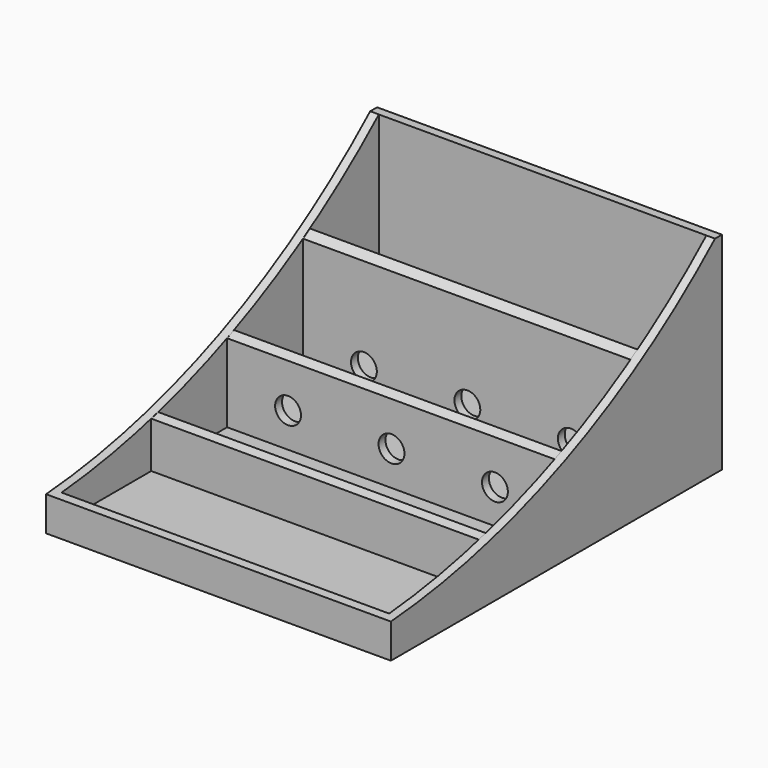
from build123d import *

# Parameters (mm, degrees)
F0_W          = 254
F0_H          = 304.8
F0_W_2        = 241.3
F0_H_2        = 292.1
F1_DEPTH      = 152.4
F3_DEPTH      = 254
F4_W          = 241.3
F4_H          = 292.1
F5_DEPTH      = 6.35
F7_END_RADIUS = 508
F6_W          = 241.3
F6_H          = 6.35
F7_REACH      = 387.4345381711
F9_DEPTH      = 12.7
F10_R         = 9.525
F11_DEPTH     = 99.06
F12_R         = 9.525
F13_DEPTH     = 25.4


# Not quite as in the source:
# - a feature names something its author has since deleted; it is built from what else it names


with BuildPart() as f1:
    # F0 (on Top) → F1 (new body)
    with BuildSketch(Plane.XY):
        with Locations((-0.4414357245, 28.0319261778)):
            Rectangle(F0_W, F0_H)
        with Locations((-0.4414357245, 28.0319261778)):
            Rectangle(F0_W_2, F0_H_2, mode=Mode.SUBTRACT)
    extrude(amount=F1_DEPTH)

    # F2 (on face) → F3 (cut, through all)
    with BuildSketch(Plane.YZ.offset(126.5585642755)):
        with BuildLine():
            Line((-124.3680738222, 152.4), (-124.3680738222, 25.4))
            ThreePointArc((-124.3680738222, 25.4), (35.2650996978, 64.440792228), (174.0819261778, 152.4))
            Line((174.0819261778, 152.4), (-124.3680738222, 152.4))
        make_face()
    extrude(amount=-F3_DEPTH, mode=Mode.SUBTRACT)

    # F8 (on face) → F9 (cut)
    with BuildSketch(Plane(origin=(0, 180.4319261778, 0), x_dir=(-1, 0, 0), z_dir=(0, 1, 0))):
        with BuildLine():
            Line((63.9414357245, 44.45), (-63.0585642755, 44.45))
            ThreePointArc((-63.0585642755, 44.45), (-82.1085642755, 25.4), (-63.0585642755, 6.35))
            Line((-63.0585642755, 6.35), (63.9414357245, 6.35))
            ThreePointArc((63.9414357245, 6.35), (82.9914357245, 25.4), (63.9414357245, 44.45))
        make_face()
    extrude(amount=-F9_DEPTH, mode=Mode.SUBTRACT)

    # F12 (on face) → F13 (cut)
    with BuildSketch(Plane(origin=(0, 40.7319261778, 0), x_dir=(-1, 0, 0), z_dir=(0, 1, 0))):
        with Locations((0, 31.75)):
            Circle(F12_R)
        with Locations((-76.2, 31.75)):
            Circle(F12_R)
        with Locations((76.2, 31.75)):
            Circle(F12_R)
    extrude(amount=-F13_DEPTH, mode=Mode.SUBTRACT)


with BuildPart() as f5:
    # F4 (on face) → F5 (new body)
    with BuildSketch(Plane(origin=(0, 0, 0), x_dir=(1, 0, 0), z_dir=(0, 0, -1))):
        with Locations((-0.4414357245, -28.0319261778)):
            Rectangle(F4_W, F4_H)
    extrude(amount=-F5_DEPTH)


with BuildPart() as f7:
    f7_end = (Plane(origin=(-0.4414357245, -163.6449236636, 531.8793471273), x_dir=(0, 0, 1), z_dir=(1, 0, 0)) * Cylinder(F7_END_RADIUS, 1624.9156633008, mode=Mode.PRIVATE)).faces().sort_by_distance((122.4388870733, 35.2650996978, 64.440792228))[0]
    # F6 (on face) → F7 (new body, up to the whole of a round face its end follows)
    with BuildSketch(Plane.XY.offset(6.35)):
        with Locations((-0.4414357245, 37.5569261778)):
            Rectangle(F6_W, F6_H)
    f7_long = extrude(amount=F7_REACH, mode=Mode.PRIVATE)
    add(split(f7_long, bisect_by=f7_end, keep=Keep.TOP, mode=Mode.PRIVATE))


with BuildPart() as f7b:
    f7_2_end = (Plane(origin=(-0.4414357245, -163.6449236636, 531.8793471273), x_dir=(0, 0, 1), z_dir=(1, 0, 0)) * Cylinder(F7_END_RADIUS, 1624.9156633008, mode=Mode.PRIVATE)).faces().sort_by_distance((122.4388870733, 35.2650996978, 64.440792228))[0]
    # F6 (on face) → F7, piece 2 (new body, up to the whole of a round face its end follows)
    with BuildSketch(Plane.XY.offset(6.35)):
        with Locations((-0.4414357245, 107.4069261778)):
            Rectangle(F6_W, F6_H)
    f7_2_long = extrude(amount=F7_REACH, mode=Mode.PRIVATE)
    add(split(f7_2_long, bisect_by=f7_2_end, keep=Keep.TOP, mode=Mode.PRIVATE))


with BuildPart() as f7c:
    f7_3_end = (Plane(origin=(-0.4414357245, -163.6449236636, 531.8793471273), x_dir=(0, 0, 1), z_dir=(1, 0, 0)) * Cylinder(F7_END_RADIUS, 1624.9156633008, mode=Mode.PRIVATE)).faces().sort_by_distance((122.4388870733, 35.2650996978, 64.440792228))[0]
    # F6 (on face) → F7, piece 3 (new body, up to the whole of a round face its end follows)
    with BuildSketch(Plane.XY.offset(6.35)):
        with Locations((-0.4414357245, -32.2930738222)):
            Rectangle(F6_W, F6_H)
    f7_3_long = extrude(amount=F7_REACH, mode=Mode.PRIVATE)
    add(split(f7_3_long, bisect_by=f7_3_end, keep=Keep.TOP, mode=Mode.PRIVATE))


with BuildPart() as f11_tool:
    # F10 (on face) → F11 (new body)
    with BuildSketch(Plane(origin=(0, 110.5819261778, 0), x_dir=(-1, 0, 0), z_dir=(0, 1, 0))):
        with Locations((76.2, 31.75)):
            Circle(F10_R)
        with Locations((0, 31.75)):
            Circle(F10_R)
        with Locations((-76.2, 31.75)):
            Circle(F10_R)
    extrude(amount=-F11_DEPTH)


with BuildPart() as f7_1:
    add(f7.part)

    # F11: cut by f11_tool
    add(f11_tool.part, mode=Mode.SUBTRACT)


with BuildPart() as f7b_1:
    add(f7b.part)

    # F11: cut by f11_tool
    add(f11_tool.part, mode=Mode.SUBTRACT)


solid = Compound([f1.part, f5.part, f7c.part, f7_1.part, f7b_1.part])
